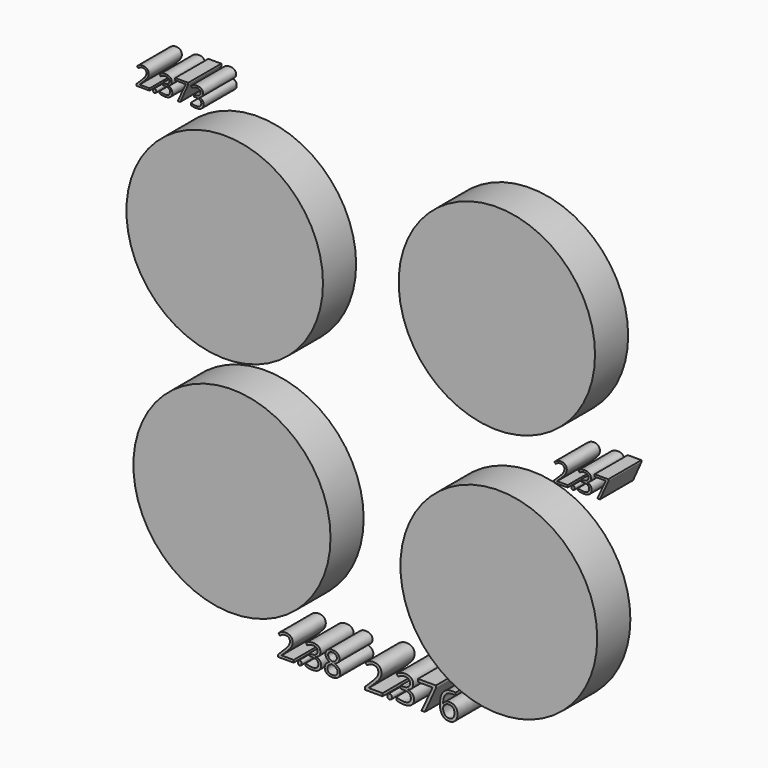
from build123d import *

# Parameters (mm, degrees)
F0_R           = 30.1371
F0_R_2         = 30.099
F0_R_3         = 30.226
F0_R_4         = 30.1752
F0_TEXT_SIZE   = 8.8148569274
F0_TEXT_SIZE_2 = 8.381344378
F0_TEXT_SIZE_3 = 10.1154152718
F0_TEXT_SIZE_4 = 11.5604657266
F1_DEPTH       = 12.7


# Not quite as in the source:
# - Text() gives the source's letters only with a copy of the font that has no kerning and outlines rounded to 1/6400 em; it was checked with that copy


with BuildPart() as f1:
    # F0 (on Front) → F1 (new body)
    with BuildSketch(Plane.XZ):
        with Locations((-42.4295477569, 30.7109095156)):
            Circle(F0_R)
        with Locations((41.0152301192, 38.5906808078)):
            Circle(F0_R_2)
        with Locations((-40.2070470154, -37.1763631701)):
            Circle(F0_R_3)
        with Locations((41.6213646531, -37.782497704)):
            Circle(F0_R_4)
        with Locations((58.1607185304, 0)):
            Text('2.37', F0_TEXT_SIZE, font='Open Sans', text_align=(TextAlign.LEFT, TextAlign.BOTTOM))
        with Locations((-69.8136687279, 65.4438063502)):
            Text('2.373', F0_TEXT_SIZE_2, font='Open Sans', text_align=(TextAlign.LEFT, TextAlign.BOTTOM))
        with Locations((-26.5312753618, -74.5997056365)):
            Text('2.38', F0_TEXT_SIZE_3, font='Open Sans', text_align=(TextAlign.LEFT, TextAlign.BOTTOM))
        with Locations((0, -74.807792902)):
            Text('2.376', F0_TEXT_SIZE_4, font='Open Sans', text_align=(TextAlign.LEFT, TextAlign.BOTTOM))
    extrude(amount=F1_DEPTH)


solid = f1.part
